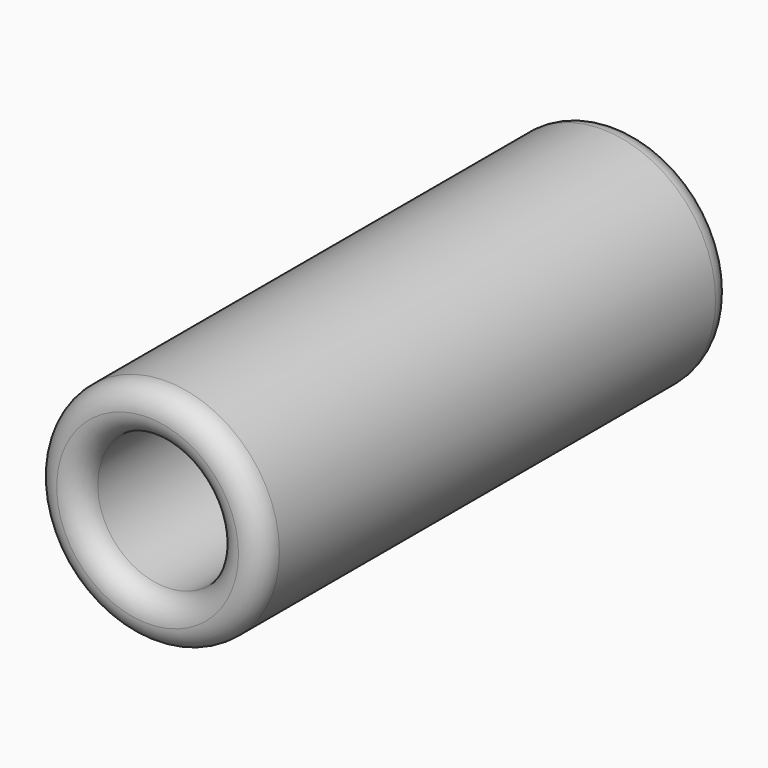
from build123d import *

# Parameters (mm, degrees)
F0_R     = 25
F0_R_2   = 15
F1_DEPTH = 130
F2_R     = 4.99999


# Not quite as in the source:
# - a fillet or chamfer is up to 0.001 mm smaller than in the source, because OpenCascade refuses the exact size


with BuildPart() as f1:
    # F0 (on Front) → F1 (new body)
    with BuildSketch(Plane.XZ):
        Circle(F0_R)
        Circle(F0_R_2, mode=Mode.SUBTRACT)
    extrude(amount=-F1_DEPTH)

    # F2 (radius 5 in the source; OpenCascade refuses exactly that, so slightly less here)
    f2_edges = [f1.edges().sort_by_distance(p)[0] for p in [
        (-15, 0, 0),
        (-25, 0, 0),
        (25, 65, 0),
        (-25, 130, 0),
        (-15, 130, 0),
    ]]
    fillet(f2_edges, radius=F2_R)


solid = f1.part
